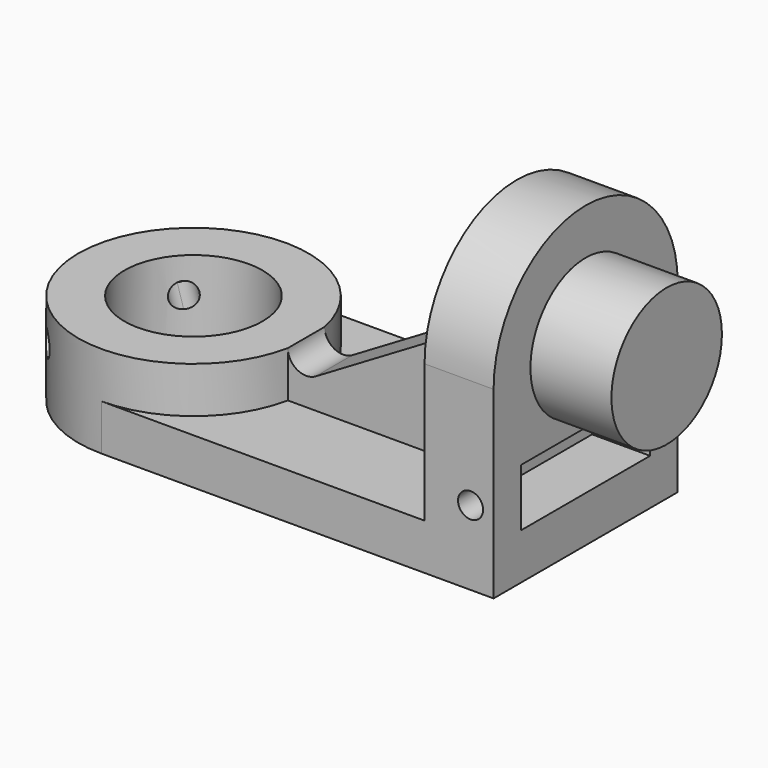
from build123d import *

# Parameters (mm, degrees)
F0_R           = 15.875
F0_R_2         = 9.525
F1_DEPTH       = 12.7
F5_DEPTH       = 25.4
F7_DEPTH       = 25.4
F9_DEPTH       = 6.35
F11_W          = 31.75
F11_H          = 19.05
F12_DEPTH      = 9.525
F14_END_RADIUS = 15.875
F13_W          = 3.175
F13_H          = 19.05
F14_REACH      = 79.7657711337
F16_DEPTH      = 25.4
F17_R          = 9.525
F18_DEPTH      = 11.176
F19_W          = 22.225
F19_H          = 7.9375
F20_DEPTH      = 8.001
F21_R          = 1.7272
F22_DEPTH      = 101.6


with BuildPart() as f1:
    # F0 (on Top) → F1 (new body)
    with BuildSketch(Plane.XY):
        Circle(F0_R)
        Circle(F0_R_2, mode=Mode.SUBTRACT)
    extrude(amount=F1_DEPTH)

    # F4 (on face) → F5 (cut)
    with BuildSketch(Plane(origin=(0, 0, 0), x_dir=(-0.7071067812, 0.7071067812, 0), z_dir=(0.7071067812, 0.7071067812, 0))):
        with BuildLine():
            ThreePointArc((0, 6.1468), (1.2213148325, 6.6526851675), (1.7272, 7.874))
            ThreePointArc((1.7272, 7.874), (1.2213148325, 9.0953148325), (0, 9.6012))
            Line((0, 9.6012), (0, 6.1468))
        make_face()
        with BuildLine():
            Line((0, 6.1468), (0, 9.6012))
            ThreePointArc((0, 9.6012), (-1.7272, 7.874), (0, 6.1468))
        make_face()
    extrude(amount=-F5_DEPTH, mode=Mode.SUBTRACT)

    # F6 (on face) → F7 (cut)
    with BuildSketch(Plane(origin=(0, 0, 0), x_dir=(-0.7071067812, -0.7071067812, 0), z_dir=(-0.7071067812, 0.7071067812, 0))):
        with BuildLine():
            ThreePointArc((0, 6.1468), (1.2213148325, 6.6526851675), (1.7272, 7.874))
            ThreePointArc((1.7272, 7.874), (1.2213148325, 9.0953148325), (0, 9.6012))
            Line((0, 9.6012), (0, 6.1468))
        make_face()
        with BuildLine():
            Line((0, 6.1468), (0, 9.6012))
            ThreePointArc((0, 9.6012), (-1.7272, 7.874), (0, 6.1468))
        make_face()
    extrude(amount=F7_DEPTH, mode=Mode.SUBTRACT)

    # F8 (on face) → F9 (join)
    with BuildSketch(Plane(origin=(0, 0, 0), x_dir=(1, 0, 0), z_dir=(0, 0, -1))):
        with BuildLine():
            Line((54.102, 15.875), (0, 15.875))
            ThreePointArc((0, 15.875), (11.2253201513, 11.2253201513), (15.875, 0))
            ThreePointArc((15.875, 0), (11.2253201513, -11.2253201513), (0, -15.875))
            Line((0, -15.875), (54.102, -15.875))
            Line((54.102, -15.875), (54.102, 15.875))
        make_face()
    extrude(amount=-F9_DEPTH)

    # F11 (on offset) → F12 (join)
    with BuildSketch(Plane.YZ.offset(54.102)):
        with Locations((0, 15.875)):
            Rectangle(F11_W, F11_H)
        with BuildLine():
            ThreePointArc((15.875, 25.4), (0, 41.275), (-15.875, 25.4))
            Line((-15.875, 25.4), (15.875, 25.4))
        make_face()
    extrude(amount=-F12_DEPTH)

    f14_end = (Plane(origin=(0, 0, 6.35), x_dir=(-1, 0, 0), z_dir=(0, 0, -1)) * Cylinder(F14_END_RADIUS, 333.9846154871, mode=Mode.PRIVATE)).faces().sort_by_distance((-15.875, 0, 6.35))[0]
    # F13 (on face) → F14 (join, up to the whole of a round face its end follows)
    with BuildSketch(Plane(origin=(44.577, 0, 0), x_dir=(0, -1, 0), z_dir=(-1, 0, 0))):
        with Locations((-1.5875, 15.875)):
            Rectangle(F13_W, F13_H)
        with Locations((1.5875, 15.875)):
            Rectangle(F13_W, F13_H)
    f14_long = extrude(amount=F14_REACH, mode=Mode.PRIVATE)
    add(split(f14_long, bisect_by=f14_end, keep=Keep.ALL, mode=Mode.PRIVATE).solids().sort_by_distance((44.577, 0, 15.875))[0])

    # F15 (on face) → F16 (cut)
    with BuildSketch(Plane.XZ.offset(3.175)):
        with BuildLine():
            Line((19.3865235489, 10.5133005292), (44.577, 25.4))
            Line((44.577, 25.4), (15.5542598667, 25.4))
            Line((15.5542598667, 25.4), (15.5542598667, 12.7))
            ThreePointArc((15.5542598667, 12.7), (16.8354409267, 10.4938778646), (19.3865235489, 10.5133005292))
        make_face()
    extrude(amount=-F16_DEPTH, mode=Mode.SUBTRACT)

    # F17 (on face) → F18 (join)
    with BuildSketch(Plane.YZ.offset(54.102)):
        with Locations((0, 25.4)):
            Circle(F17_R)
    extrude(amount=F18_DEPTH)

    # F19 (on face) → F20 (cut)
    with BuildSketch(Plane.YZ.offset(54.102)):
        with Locations((0, 10.31875)):
            Rectangle(F19_W, F19_H)
    extrude(amount=-F20_DEPTH, mode=Mode.SUBTRACT)

    # F21 (on face) → F22 (cut)
    with BuildSketch(Plane.XZ.offset(15.875)):
        with Locations((50.927, 10.287)):
            Circle(F21_R)
    extrude(amount=-F22_DEPTH, mode=Mode.SUBTRACT)


solid = f1.part
